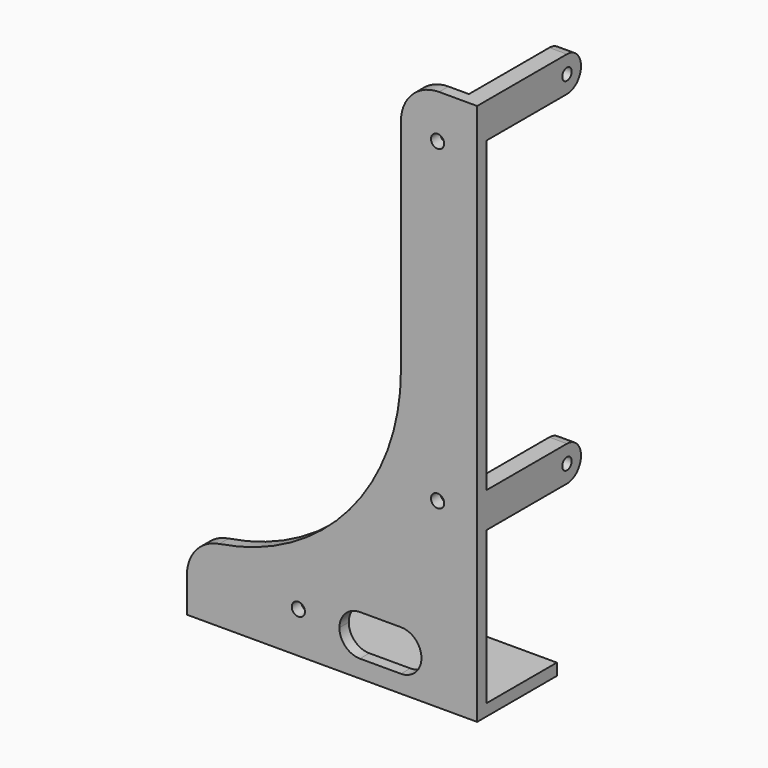
from build123d import *

# Parameters (mm, degrees)
F0_R        = 2
F1_DEPTH    = 6
F2_DEPTH    = 93
F4_DEPTH    = 25
F3_R        = 1.75
F5_DEPTH    = 4.001
F6_W        = 73
F6_H        = 161
F6_R        = 2.25
F7_DEPTH    = 4.001
F8_T4_DEPTH = 4
F9_R        = 13


# Not quite as in the source:
# - a fillet or chamfer that OpenCascade refuses, or shapes differently, is made with other operations: its cross-section is extruded or revolved along the edge and cut away or added


with BuildPart() as f1:
    # F0 (on Right) → F1 (new body)
    with BuildSketch(Plane.YZ):
        Polygon((-4.3, 0), (-34.3, 0), (-34.3, 52), (-34.3, 64), (-34.3, 169), (-34.3, 181), (-38.3, 181), (-38.3, -4), (-4.3, -4), align=None)
        with BuildLine():
            Line((-34.3, 181), (-34.3, 169))
            Line((-34.3, 169), (0, 169))
            ThreePointArc((0, 169), (-6, 174.9999999833), (-3.34e-08, 181))
            Line((-3.34e-08, 181), (-34.3, 181))
        make_face()
        with BuildLine():
            Line((-34.3, 64), (-34.3, 52))
            Line((-34.3, 52), (-5.41e-08, 52))
            ThreePointArc((-5.41e-08, 52), (-6, 58.0000000477), (4.13e-08, 64))
            Line((4.13e-08, 64), (-34.3, 64))
        make_face()
        with BuildLine():
            ThreePointArc((-3.34e-08, 181), (-6, 174.9999999833), (0, 169))
            ThreePointArc((0, 169), (4.2426406871, 170.7573593129), (6, 175))
            ThreePointArc((6, 175), (4.2426406753, 179.2426406989), (-3.34e-08, 181))
        make_face()
        with Locations((0, 175)):
            Circle(F0_R, mode=Mode.SUBTRACT)
        with BuildLine():
            ThreePointArc((4.13e-08, 64), (-6, 58.0000000477), (-5.41e-08, 52))
            ThreePointArc((-5.41e-08, 52), (4.242640668, 53.7573592937), (6, 58))
            ThreePointArc((6, 58), (4.2426407017, 62.2426406725), (4.13e-08, 64))
        make_face()
        with Locations((0, 58)):
            Circle(F0_R, mode=Mode.SUBTRACT)
    extrude(amount=F1_DEPTH)

    # F0 (on Right) → F2 (join)
    with BuildSketch(Plane.YZ):
        Polygon((-4.3, 0), (-34.3, 0), (-34.3, 52), (-34.3, 64), (-34.3, 169), (-34.3, 181), (-38.3, 181), (-38.3, -4), (-4.3, -4), align=None)
    extrude(amount=-F2_DEPTH)

    # F0 (on Right) → F4 (join)
    with BuildSketch(Plane.YZ):
        Polygon((-4.3, 0), (-34.3, 0), (-34.3, 52), (-34.3, 64), (-34.3, 169), (-34.3, 181), (-38.3, 181), (-38.3, -4), (-4.3, -4), align=None)
    extrude(amount=-F4_DEPTH)

    # F3 (on face) → F5 (cut, through all)
    with BuildSketch(Plane.XY):
        with Locations((-89, -27.8)):
            Circle(F3_R)
        with Locations((-69, -27.8)):
            Circle(F3_R)
    extrude(amount=-F5_DEPTH, mode=Mode.SUBTRACT)

    # F6 (on face) → F7 (cut, through all)
    with BuildSketch(Plane(origin=(0, -34.3, 0), x_dir=(-1, 0, 0), z_dir=(0, 1, 0))):
        with Locations((56.5, 100.5)):
            Rectangle(F6_W, F6_H)
        with BuildLine():
            ThreePointArc((20, 2), (24.9497474683, 4.0502525317), (27, 9))
            ThreePointArc((27, 9), (24.9497474683, 13.9497474683), (20, 16))
            ThreePointArc((20, 16), (13, 9), (20, 2))
        make_face()
        with BuildLine():
            ThreePointArc((34, 2), (29.0502525317, 4.0502525317), (27, 9))
            ThreePointArc((27, 9), (24.9497474683, 4.0502525317), (20, 2))
            Line((20, 2), (34, 2))
        make_face()
        with BuildLine():
            ThreePointArc((20, 16), (24.9497474683, 13.9497474683), (27, 9))
            ThreePointArc((27, 9), (29.0502525317, 13.9497474683), (34, 16))
            Line((34, 16), (20, 16))
        make_face()
        with BuildLine():
            ThreePointArc((34, 16), (29.0502525317, 13.9497474683), (27, 9))
            ThreePointArc((27, 9), (29.0502525317, 4.0502525317), (34, 2))
            ThreePointArc((34, 2), (38.9497474683, 4.0502525317), (41, 9))
            ThreePointArc((41, 9), (38.9497474683, 13.9497474683), (34, 16))
        make_face()
        with Locations((7.5, 166)):
            Circle(F6_R)
        with Locations((7.5, 58)):
            Circle(F6_R)
        with Locations((55, 10)):
            Circle(F6_R)
    extrude(amount=-F7_DEPTH, mode=Mode.SUBTRACT)

    # F8: fillet of radius 73.1506709399 on 1 edges, made by hand


with BuildPart() as f8_tool2:
    # F8_s3 → F8_t4 (new body)
    with BuildSketch(Plane.XZ.offset(34.3)):
        with BuildLine():
            ThreePointArc((-93.1506709399, 20), (-41.42533547, 41.42533547), (-20, 93.1506709399))
            Line((-20, 93.1506709399), (-20, 20))
            Line((-20, 20), (-93.1506709399, 20))
        make_face()
    extrude(amount=F8_T4_DEPTH)

    split(bisect_by=Plane.YZ.offset(-93), keep=Keep.TOP)


with BuildPart() as f1_1:
    add(f1.part)

    # F8_t1: union F8_tool2
    add(f8_tool2.part)

    # F9
    f9_edges = [f1_1.edges().sort_by_distance(p)[0] for p in [
        (-20, -36.3, 181),
        (-93, -36.3, 20.000155),
    ]]
    fillet(f9_edges, radius=F9_R)


solid = f1_1.part
